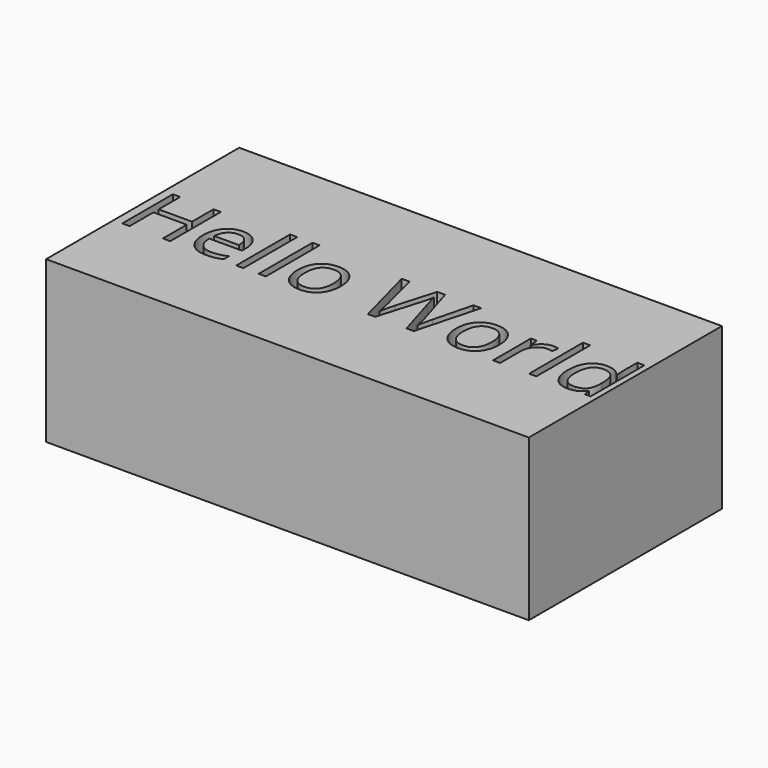
from build123d import *

# Parameters (mm, degrees)
F0_W         = 76.2
F0_H         = 25.4
F1_DEPTH     = 38.1
F2_TEXT_SIZE = 13.9776440241
F3_DEPTH     = 25.4


# Not quite as in the source:
# - Text() gives the source's letters only with a copy of the font that has no kerning and outlines rounded to 1/6400 em; it was checked with that copy


with BuildPart() as f1:
    # F0 (on Front) → F1 (new body)
    with BuildSketch(Plane.XZ):
        with Locations((38.1, 12.7)):
            Rectangle(F0_W, F0_H)
    extrude(amount=F1_DEPTH)

    # F2 (on face) → F3 (cut)
    with BuildSketch(Plane.XY.offset(25.4)):
        with Locations((0, -24.7767738923)):
            Text('Hello World', F2_TEXT_SIZE, font='Open Sans', text_align=(TextAlign.LEFT, TextAlign.BOTTOM))
    extrude(amount=-F3_DEPTH, mode=Mode.SUBTRACT)


solid = f1.part
